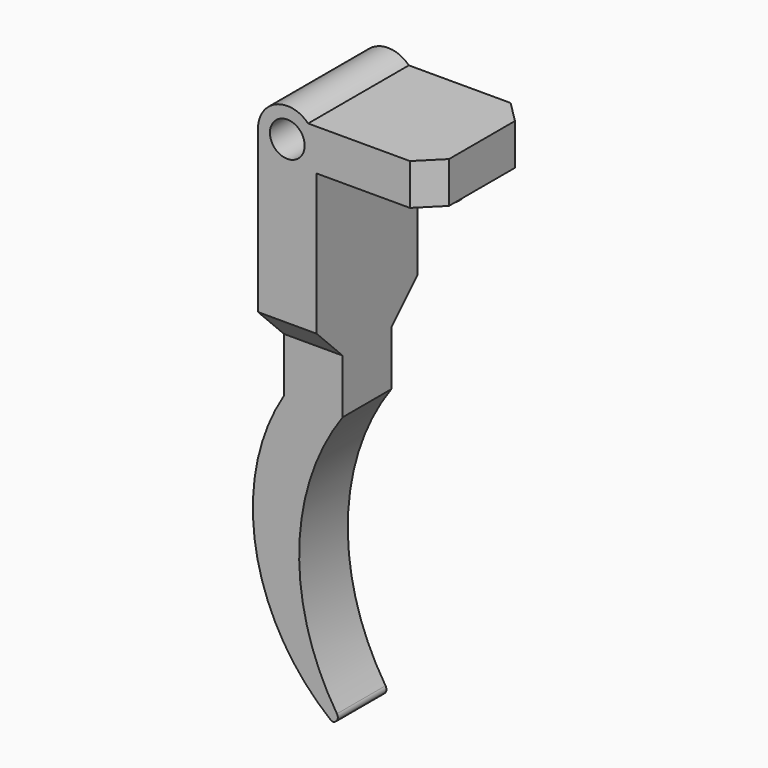
from build123d import *

# Parameters (mm, degrees)
F0_R        = 1.6
F1_DEPTH    = 5.8
F0_W        = 5.4
F0_H        = 5
F2_DEPTH    = 2.8
F3_SIZE     = 2.99999
F4_R        = 1.5
F5_DEPTH    = 2
F6_R        = 1
F7_T1_DEPTH = 6.481505829
F7_T3_DEPTH = 10.3311661503
F8_SIZE     = 2


# Not quite as in the source:
# - a fillet or chamfer that OpenCascade refuses, or shapes differently, is made with other operations: its cross-section is extruded or revolved along the edge and cut away or added
# - a fillet or chamfer is up to 0.001 mm smaller than in the source, because OpenCascade refuses the exact size


with BuildPart() as f1:
    # F0 (on Front) → F1 (new body, symmetric)
    with BuildSketch(Plane.XZ):
        with BuildLine():
            ThreePointArc((1.9183326093, -1.9), (2.4969479415, -1.0272540958), (2.7, 0))
            ThreePointArc((2.7, 0), (2.4969479415, 1.0272540958), (1.9183326093, 1.9))
            ThreePointArc((1.9183326093, 1.9), (-1.0272540958, 2.4969479415), (-2.7, 0))
            ThreePointArc((-2.7, 0), (-1.0272540958, -2.4969479415), (1.9183326093, -1.9))
        make_face()
        Circle(F0_R, mode=Mode.SUBTRACT)
        with BuildLine():
            ThreePointArc((1.9183326093, 1.9), (2.4969479415, 1.0272540958), (2.7, 0))
            ThreePointArc((2.7, 0), (2.4969479415, -1.0272540958), (1.9183326093, -1.9))
            Line((1.9183326093, -1.9), (2.7, -1.9))
            Line((2.7, -1.9), (13.3, -1.9))
            Line((13.3, -1.9), (13.3, 1.9))
            Line((13.3, 1.9), (1.9183326093, 1.9))
        make_face()
        with BuildLine():
            Line((2.7, -1.9), (1.9183326093, -1.9))
            ThreePointArc((1.9183326093, -1.9), (-1.0272540958, -2.4969479415), (-2.7, 0))
            Line((-2.7, 0), (-2.7, -17.9))
            Line((-2.7, -17.9), (2.7, -17.9))
            Line((2.7, -17.9), (2.7, -1.9))
        make_face()
    extrude(amount=F1_DEPTH, both=True)

    # F0 (on Front) → F2 (join, symmetric)
    with BuildSketch(Plane.XZ):
        with BuildLine():
            Line((2.7, -22.9), (-2.7, -22.9))
            ThreePointArc((-2.7, -22.9), (-5.2874639524, -36.2425936556), (1.7, -47.9))
            Line((1.7, -47.9), (2.7, -47.9))
            ThreePointArc((2.7, -47.9), (-1.3071443155, -35.4), (2.7, -22.9))
        make_face()
        with Locations((0, -20.4)):
            Rectangle(F0_W, F0_H)
    extrude(amount=F2_DEPTH, both=True)

    # F3 (size 3 in the source; OpenCascade refuses exactly that, so slightly less here)
    f3_edges = [f1.edges().sort_by_distance(p)[0] for p in [
        (0, -5.8, -17.9),
        (0, 5.8, -17.9),
    ]]
    chamfer(f3_edges, length=F3_SIZE)

    # F4 (on face) → F5 (join)
    with BuildSketch(Plane(origin=(0, 0, -1.9), x_dir=(1, 0, 0), z_dir=(0, 0, -1))):
        with Locations((10.1, 0)):
            Circle(F4_R)
    extrude(amount=F5_DEPTH)

    # F6
    f6_edges = [f1.edges().sort_by_distance(p)[0] for p in [
        (8.6, 0, -3.9),
    ]]
    fillet(f6_edges, radius=F6_R)

    # F7: fillet of radius 0.5 on 2 edges, made by hand

    # F7_s2 → F7_t1 (cut)
    with BuildSketch(Plane.XZ.offset(-3.2407529145)):
        with BuildLine():
            ThreePointArc((1.8739659479, -47.9), (1.7085587408, -47.871847916), (1.561777764, -47.7905618233))
            ThreePointArc((1.561777764, -47.7905618233), (1.6307619466, -47.8454412332), (1.7, -47.9))
            Line((1.7, -47.9), (1.8739659479, -47.9))
        make_face()
    extrude(amount=F7_T1_DEPTH, mode=Mode.SUBTRACT)

    # F7_s4 → F7_t3 (cut)
    with BuildSketch(Plane.XZ.offset(-5.1655830752)):
        with BuildLine():
            ThreePointArc((2.1728369726, -47.1272727273), (2.1932913064, -47.6383656473), (1.7537667699, -47.9))
            Line((1.7537667699, -47.9), (2.7, -47.9))
            ThreePointArc((2.7, -47.9), (2.4322155262, -47.5165036692), (2.1728369726, -47.1272727273))
        make_face()
    extrude(amount=F7_T3_DEPTH, mode=Mode.SUBTRACT)

    # F8
    f8_edges = [f1.edges().sort_by_distance(p)[0] for p in [
        (13.3, -5.8, 0),
        (13.3, 5.8, 0),
    ]]
    chamfer(f8_edges, length=F8_SIZE)


solid = f1.part
